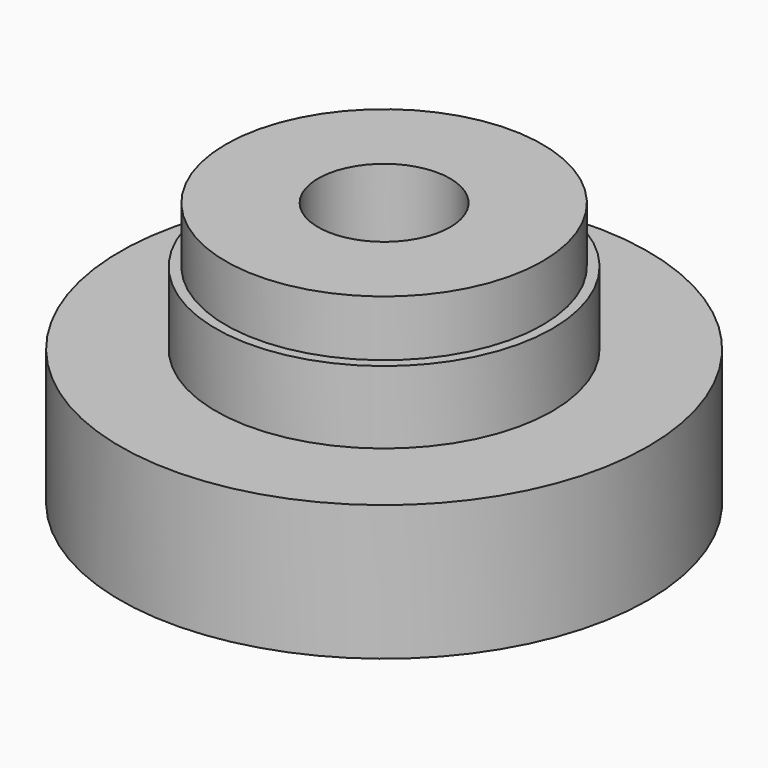
from build123d import *

# Parameters (mm, degrees)
F0_R     = 20
F1_DEPTH = 6
F2_DEPTH = 4.25
F3_R     = 12.75
F4_DEPTH = 5.5
F5_R     = 12
F6_DEPTH = 4.25
F7_R     = 5
F8_DEPTH = 73
F9_DEPTH = 20.001


# Not quite as in the source:
# - an extrude ends at something that could not be found from the text; its depth is read off the source's solid


with BuildPart() as f1:
    # F0 (on Top) → F1 (new body)
    with BuildSketch(Plane.XY):
        Circle(F0_R)
    extrude(amount=F1_DEPTH)

    # F2 (add): a face of the model
    f2_faces = [f1.faces().sort_by_distance(p)[0] for p in [
        (0, 0, 6),
    ]]
    extrude(f2_faces, amount=F2_DEPTH)

    # F3 (on face) → F4 (join)
    with BuildSketch(Plane.XY.offset(10.25)):
        Circle(F3_R)
    extrude(amount=F4_DEPTH)

    # F5 (on face) → F6 (join)
    with BuildSketch(Plane.XY.offset(15.75)):
        Circle(F5_R)
    extrude(amount=F6_DEPTH)

    # F7 (on face) → F8 (cut, through all)
    with BuildSketch(Plane.XY.offset(20)):
        Circle(F7_R)
    extrude(amount=F8_DEPTH, mode=Mode.SUBTRACT)

    # F7 (on face) → F9 (cut, through all)
    with BuildSketch(Plane.XY.offset(20)):
        Circle(F7_R)
    extrude(amount=-F9_DEPTH, mode=Mode.SUBTRACT)


solid = f1.part
